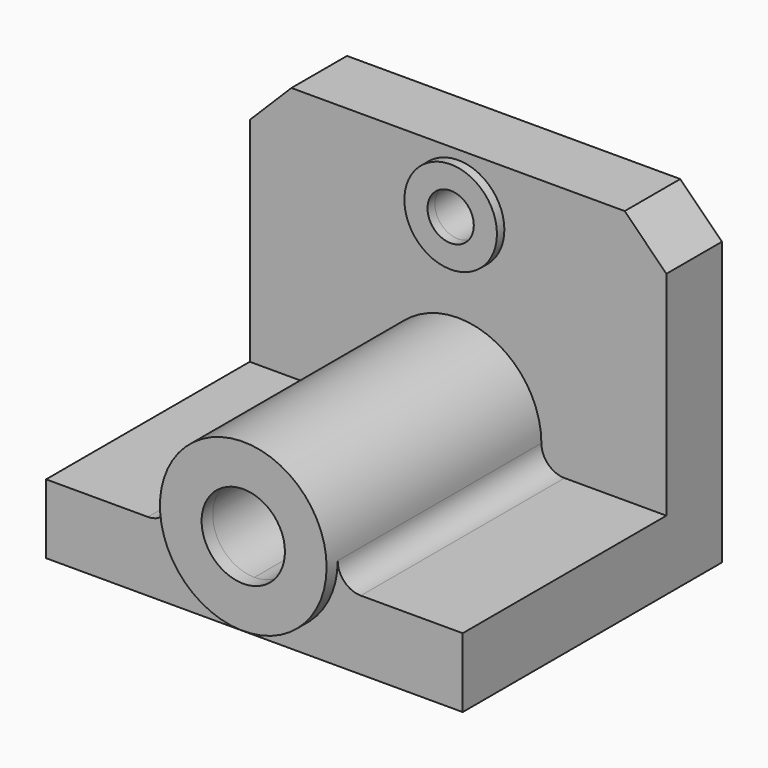
from build123d import *

# Parameters (mm, degrees)
F1_DEPTH    = 70
F2_T1_DEPTH = 70
F3_T1_DEPTH = 70
F5_DEPTH    = 15
F6_SIZE     = 9
F7_R        = 9
F8_DEPTH    = 3
F9_R        = 5
F10_DEPTH   = 25
F11_R       = 10
F11_R_2     = 5
F12_DEPTH   = 2


# Not quite as in the source:
# - a fillet or chamfer that OpenCascade refuses, or shapes differently, is made with other operations: its cross-section is extruded or revolved along the edge and cut away or added


with BuildPart() as f1:
    # F0 (on Front) → F1 (new body)
    with BuildSketch(Plane.XZ):
        with BuildLine():
            Line((45, -5), (17.2916164658, -5))
            ThreePointArc((17.2916164658, -5), (10.8166538264, -14.3874945699), (0, -18))
            Line((0, -18), (0, -20))
            Line((0, -20), (45, -20))
            Line((45, -20), (45, -5))
        make_face()
        with BuildLine():
            ThreePointArc((17.2916164658, -5), (17.8220242451, -2.5249657043), (18, 0))
            ThreePointArc((18, 0), (-2.5249657043, 17.8220242451), (-17.2916164658, -5))
            ThreePointArc((-17.2916164658, -5), (-10.8166538264, -14.3874945699), (0, -18))
            ThreePointArc((0, -18), (10.8166538264, -14.3874945699), (17.2916164658, -5))
        make_face()
        with BuildLine():
            ThreePointArc((9, 0), (6.3639610307, -6.3639610307), (0, -9))
            ThreePointArc((0, -9), (-6.3639610307, 6.3639610307), (9, 0))
        make_face(mode=Mode.SUBTRACT)
        with BuildLine():
            ThreePointArc((0, -18), (-10.8166538264, -14.3874945699), (-17.2916164658, -5))
            Line((-17.2916164658, -5), (-45, -5))
            Line((-45, -5), (-45, -20))
            Line((-45, -20), (0, -20))
            Line((0, -20), (0, -18))
        make_face()
    extrude(amount=F1_DEPTH)

    # F2: fillet of radius 5 on 1 edges, made by hand

    # F2_s2 → F2_t1 (join)
    with BuildSketch(Plane.XZ):
        with BuildLine():
            ThreePointArc((-18, 0), (-19.4644660941, -3.5355339059), (-23, -5))
            Line((-23, -5), (-17.2916164658, -5))
            ThreePointArc((-17.2916164658, -5), (-17.8220242451, -2.5249657043), (-18, 0))
        make_face()
    extrude(amount=F2_T1_DEPTH)

    # F3: fillet of radius 5 on 1 edges, made by hand

    # F3_s2 → F3_t1 (join)
    with BuildSketch(Plane.XZ):
        with BuildLine():
            ThreePointArc((23, -5), (19.4644660941, -3.5355339059), (18, 0))
            ThreePointArc((18, 0), (17.8220242451, -2.5249657043), (17.2916164658, -5))
            Line((17.2916164658, -5), (23, -5))
        make_face()
    extrude(amount=F3_T1_DEPTH)

    # F4 (on Front) → F5 (join)
    with BuildSketch(Plane.XZ):
        with BuildLine():
            Line((23, -5), (45, -5))
            Line((45, -5), (45, 50))
            Line((45, 50), (-45, 50))
            Line((-45, 50), (-45, -5))
            Line((-45, -5), (-23, -5))
            ThreePointArc((-23, -5), (-19.4644660941, -3.5355339059), (-18, 0))
            ThreePointArc((-18, 0), (0, 18), (18, 0))
            ThreePointArc((18, 0), (19.4644660941, -3.5355339059), (23, -5))
        make_face()
    extrude(amount=F5_DEPTH)

    # F6
    f6_edges = [f1.edges().sort_by_distance(p)[0] for p in [
        (45, -7.5, 50),
        (-45, -7.5, 50),
    ]]
    chamfer(f6_edges, length=F6_SIZE)

    # F7 (on face) → F8 (join)
    with BuildSketch(Plane.XZ.offset(70)):
        with BuildLine():
            ThreePointArc((-18, 0), (0, -18), (18, 0))
            ThreePointArc((18, 0), (0, 18), (-18, 0))
        make_face()
        Circle(F7_R, mode=Mode.SUBTRACT)
    extrude(amount=F8_DEPTH)

    # F9 (on face) → F10 (cut)
    with BuildSketch(Plane.XZ.offset(15)):
        with Locations((0, 38)):
            Circle(F9_R)
    extrude(amount=-F10_DEPTH, mode=Mode.SUBTRACT)

    # F11 (on face) → F12 (join)
    with BuildSketch(Plane.XZ.offset(15)):
        with Locations((0, 38)):
            Circle(F11_R)
        with Locations((0, 38)):
            Circle(F11_R_2, mode=Mode.SUBTRACT)
    extrude(amount=F12_DEPTH)


solid = f1.part
